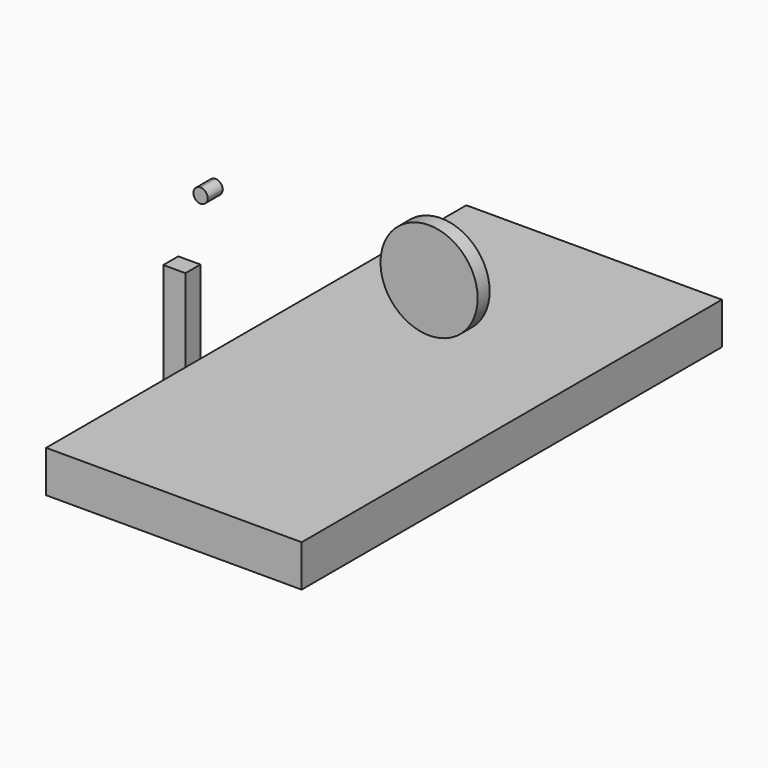
from build123d import *

# Parameters (mm, degrees)
F0_W        = 86.512580514
F0_H        = 14.1360429116
F1_DEPTH    = 88.9
F4_DEPTH    = 6.35
F5_R        = 16.4367622898
F6_DEPTH    = 5.08
F7_W        = 4.9004927278
F7_H        = 4.9005001783
F8_DEPTH    = 6.35
F9_T1_DEPTH = 19.05


# Not quite as in the source:
# - a fillet or chamfer that OpenCascade refuses, or shapes differently, is made with other operations: its cross-section is extruded or revolved along the edge and cut away or added


with BuildPart() as f1:
    # F0 (on Front) → F1 (new body)
    with BuildSketch(Plane.XZ):
        with Locations((2.1675266325, 0.5654415581)):
            Rectangle(F0_W, F0_H)
    extrude(amount=F1_DEPTH)

    # F2: F1 across plane


with BuildPart() as f1_1:
    add(f1.part)
    add(f1.part.mirror(Plane.XZ))


with BuildPart() as f4:
    # F3 (on Front) → F4 (new body)
    with BuildSketch(Plane.XZ):
        Polygon((-67.4644317088, 19.9753048493), (-67.4644317088, -43.1589859507), (-59.9484388175, -43.1589859507), (-59.9484388175, 19.9753138556), align=None)
    extrude(amount=F4_DEPTH)


with BuildPart() as f6:
    # F5 (on Front) → F6 (new body)
    with BuildSketch(Plane.XZ):
        with Locations((21.4867834002, 43.8217334449)):
            Circle(F5_R)
    extrude(amount=F6_DEPTH)


with BuildPart() as f8:
    # F7 (on Front) → F8 (new body)
    with BuildSketch(Plane.XZ):
        with Locations((-54.847843945, 44.7641350329)):
            Rectangle(F7_W, F7_H)
    extrude(amount=F8_DEPTH)

    # F9: fillet of radius 2.54 on 4 edges, made by hand

    # F9_s2 → F9_t1 (cut)
    with BuildSketch(Plane.XZ.offset(-6.35)):
        with BuildLine():
            ThreePointArc((-54.7580903089, 47.2143851221), (-56.5541415331, 46.4704363463), (-57.2980903089, 44.6743851221))
            Line((-57.2980903089, 44.6743851221), (-57.2980903089, 47.2143851221))
            Line((-57.2980903089, 47.2143851221), (-54.7580903089, 47.2143851221))
        make_face()
        with BuildLine():
            ThreePointArc((-52.3975975811, 44.6743851221), (-53.1415463569, 46.4704363463), (-54.9375975811, 47.2143851221))
            Line((-54.9375975811, 47.2143851221), (-52.3975975811, 47.2143851221))
            Line((-52.3975975811, 47.2143851221), (-52.3975975811, 44.6743851221))
        make_face()
        with BuildLine():
            ThreePointArc((-54.7580903089, 42.3138849437), (-56.5541415331, 43.0578337195), (-57.2980903089, 44.8538849437))
            Line((-57.2980903089, 44.8538849437), (-57.2980903089, 42.3138849437))
            Line((-57.2980903089, 42.3138849437), (-54.7580903089, 42.3138849437))
        make_face()
        with BuildLine():
            ThreePointArc((-54.9375975811, 42.3138849437), (-53.1415463569, 43.0578337195), (-52.3975975811, 44.8538849437))
            Line((-52.3975975811, 44.8538849437), (-52.3975975811, 42.3138849437))
            Line((-52.3975975811, 42.3138849437), (-54.9375975811, 42.3138849437))
        make_face()
    extrude(amount=F9_T1_DEPTH, mode=Mode.SUBTRACT)


solid = Compound([f1_1.part, f4.part, f6.part, f8.part])
